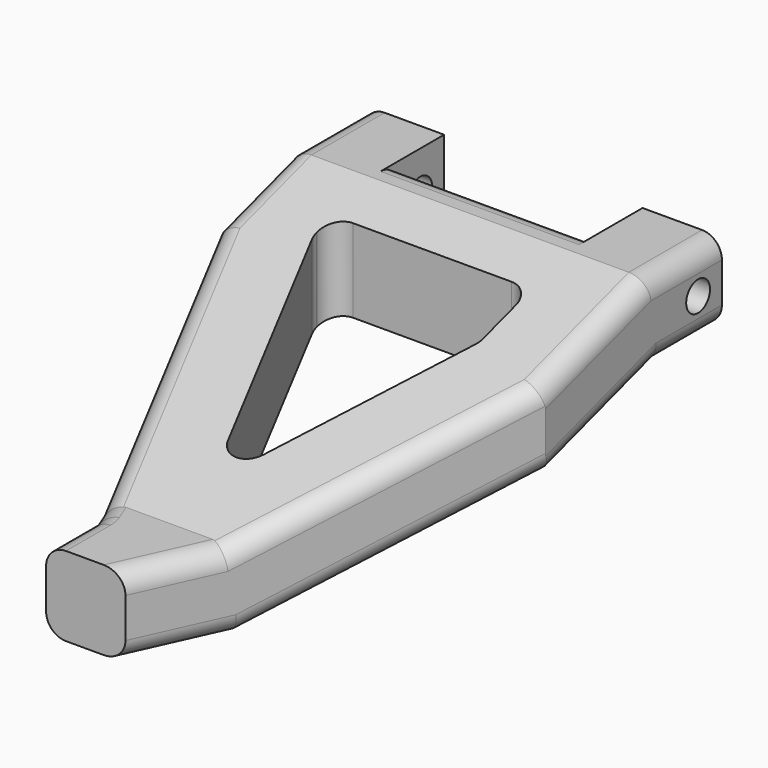
from build123d import *

# Parameters (mm, degrees)
F1_DEPTH = 127
F3_DEPTH = 627.38
F5_DEPTH = 546.1
F6_R     = 19.05
F7_DEPTH = 409.956
F8_R     = 25.39999


# Not quite as in the source:
# - a fillet or chamfer is up to 0.001 mm smaller than in the source, because OpenCascade refuses the exact size


with BuildPart() as f1:
    # F0 (on Top) → F1 (new body, symmetric)
    with BuildSketch(Plane.XY):
        with BuildLine():
            Line((228.6, 73.2671543956), (228.6, 355.6))
            Line((228.6, 355.6), (127, 355.6))
            Line((127, 355.6), (127, 279.4))
            Line((127, 279.4), (-127, 279.4))
            Line((-127, 279.4), (-127, 355.6))
            Line((-127, 355.6), (-228.6, 355.6))
            Line((-228.6, 355.6), (-228.6, 127))
            Line((-228.6, 127), (-69.3541612572, -274.8921242948))
            ThreePointArc((-69.3541612572, -274.8921242948), (-68.0185057912, -279.4860093319), (-67.5679594278, -284.2488617581))
            Line((-67.5679594278, -284.2488617581), (-67.5679594278, -355.6))
            Line((-67.5679594278, -355.6), (34.0320405722, -355.6))
            Line((34.0320405722, -355.6), (228.6, 73.2671543956))
        make_face()
        with BuildLine():
            Line((126.9999997139, 152.3999997139), (126.9999997139, 100.7287641896))
            ThreePointArc((126.9999997139, 100.7287641896), (126.4262326875, 95.3605096932), (124.7308535455, 90.2347849149))
            Line((124.7308535455, 90.2347849149), (26.9491079367, -125.2959690409))
            ThreePointArc((26.9491079367, -125.2959690409), (3.2004851004, -140.194476085), (-19.7955440656, -124.1587272294))
            Line((-19.7955440656, -124.1587272294), (-125.2137978845, 141.8875713817))
            ThreePointArc((-125.2137978845, 141.8875713817), (-126.5494533505, 146.4814564188), (-126.9999997139, 151.244308845))
            Line((-126.9999997139, 151.244308845), (-126.9999997139, 152.3999997139))
            ThreePointArc((-126.9999997139, 152.3999997139), (-119.560511956, 170.360511956), (-101.5999997139, 177.7999997139))
            Line((-101.5999997139, 177.7999997139), (101.5999997139, 177.7999997139))
            ThreePointArc((101.5999997139, 177.7999997139), (119.560511956, 170.360511956), (126.9999997139, 152.3999997139))
        make_face(mode=Mode.SUBTRACT)
    extrude(amount=F1_DEPTH, both=True)

    # F2 (on face) → F3 (cut)
    with BuildSketch(Plane.YZ.offset(228.6)):
        Polygon((-228.6, -127), (-355.6, -127), (-355.6, -25.4), (-399.7474312782, -25.4), (-399.7474312782, -182.4822723866), (403.1273424625, -182.4822723866), (403.1273424625, 126.7705559731), (355.6, 127), (355.6, 25.4), (254, 25.4), align=None)
    extrude(amount=-F3_DEPTH, mode=Mode.SUBTRACT)

    # F4 (on face) → F5 (cut)
    with BuildSketch(Plane.YZ.offset(228.6)):
        Polygon((238.3390568884, 127), (355.6, 127), (355.6, 150.2672582865), (-388.3270025253, 150.2672582865), (-355.6, -25.4), (-244.2609431116, -25.4), (42.6722074132, 65.2104685868), align=None)
    extrude(amount=-F5_DEPTH, mode=Mode.SUBTRACT)

    # F6 (on face) → F7 (cut, symmetric)
    with BuildSketch(Plane.YZ.offset(-127)):
        with Locations((317.5, 76.2)):
            Circle(F6_R)
    extrude(amount=F7_DEPTH, both=True, mode=Mode.SUBTRACT)

    # F8 (radius 25.4 in the source; OpenCascade refuses exactly that, so slightly less here)
    f8_edges = [f1.edges().sort_by_distance(p)[0] for p in [
        (156.572108, -85.496894, 24.736015),
        (228.6, 155.803106, 100.936015),
        (228.6, 296.969528, 127),
        (59.288128, -299.930472, -25.4),
        (-67.567959, -319.924431, -25.4),
        (-155.045734, -58.630472, 33.220149),
        (-228.6, 182.669528, 109.420149),
        (-228.6, 296.969528, 127),
        (-228.6, 304.8, 25.4),
        (-228.6, 190.5, 5.347368),
        (-158.148482, -50.8, -70.852632),
        (-78.525563, -251.746062, -127),
        (-67.567959, -319.924431, -127),
        (160.124628, -77.666423, -79.336765),
        (62.840648, -292.1, -127),
        (228.6, 163.633577, -3.136765),
        (228.6, 304.8, 25.4),
        (0, 279.4, 127),
        (0, 279.4, 25.4),
    ]]
    fillet(f8_edges, radius=F8_R)


solid = f1.part
